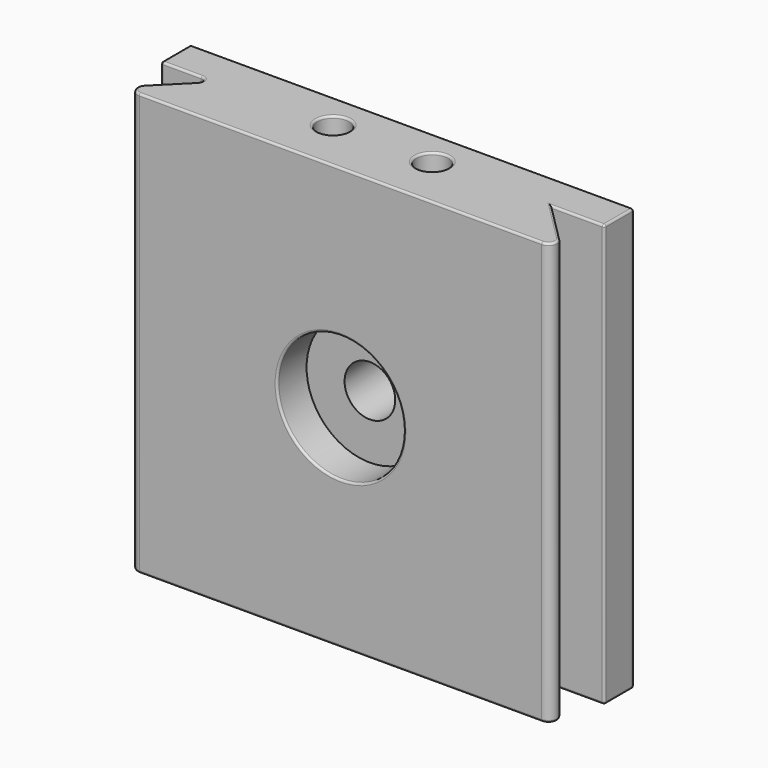
from build123d import *

# Parameters (mm, degrees)
F0_R     = 1.5
F1_DEPTH = 40
F2_R     = 2.4
F3_DEPTH = 8.001
F2_R_2   = 6
F4_DEPTH = 3.48
F5_DEPTH = 0.5
F6_R     = 0.8
F7_R     = 0.5
F8_R     = 0.2


# Not quite as in the source:
# - a feature names something its author has since deleted; it is built from what else it names


with BuildPart() as f1:
    # F0 (on Top) → F1 (new body)
    with BuildSketch(Plane.XY):
        Polygon((-13.1589230299, 2.7048220783), (-21.1589230299, 2.7048220783), (-21.1589230299, -0.2951779217), (-16.1589230299, -0.2951779217), (-21.1589230299, -5.2951779217), (-0.1589230299, -5.2951779217), (20.8410769701, -5.2951779217), (15.8410769701, -0.2951779217), (20.8410769701, -0.2951779217), (20.8410769701, 2.7048220783), (12.8410769701, 2.7048220783), (-0.1589230299, 2.7048220783), align=None)
        with Locations((-4.8589230299, -0.2951779217)):
            Circle(F0_R, mode=Mode.SUBTRACT)
        with BuildLine():
            ThreePointArc((6.0410769701, -0.2951779217), (5.6017371419, -1.3558380934), (4.5410769701, -1.7951779217))
            ThreePointArc((4.5410769701, -1.7951779217), (3.4804167983, 0.7654822501), (6.0410769701, -0.2951779217))
        make_face(mode=Mode.SUBTRACT)
    extrude(amount=F1_DEPTH)

    # F2 (on face) → F3 (cut, through all)
    with BuildSketch(Plane.XZ.offset(5.2951779217)):
        with Locations((-0.1589225605, 19.999999553)):
            Circle(F2_R)
    extrude(amount=-F3_DEPTH, mode=Mode.SUBTRACT)

    # F2 (on face) → F4 (cut)
    with BuildSketch(Plane.XZ.offset(5.2951779217)):
        with Locations((-0.1589225605, 19.999999553)):
            Circle(F2_R_2)
        with Locations((-0.1589225605, 19.999999553)):
            Circle(F2_R, mode=Mode.SUBTRACT)
    extrude(amount=-F4_DEPTH, mode=Mode.SUBTRACT)

    # F5 (add): a face of the model
    f5_faces = [f1.faces().sort_by_distance(p)[0] for p in [
        (20.2610769701, 2.7048220783, 20),
    ]]
    extrude(f5_faces, amount=F5_DEPTH)

    # F6
    f6_edges = [f1.edges().sort_by_distance(p)[0] for p in [
        (20.841077, -5.295178, 20),
        (-21.158923, -5.295178, 20),
    ]]
    fillet(f6_edges, radius=F6_R)

    # F7
    f7_edges = [f1.edges().sort_by_distance(p)[0] for p in [
        (-16.158923, -0.295178, 20),
    ]]
    fillet(f7_edges, radius=F7_R)

    # F8
    f8_edges = [f1.edges().sort_by_distance(p)[0] for p in [
        (-18.402857, -2.539112, 40),
        (-16.90409, -0.603836, 40),
        (-19.966656, -4.801325, 40),
        (-19.262476, -0.295178, 40),
        (-0.158923, -5.295178, 40),
        (-21.158923, 1.454822, 40),
        (19.64881, -4.801325, 40),
        (-0.158923, 3.204822, 40),
        (17.658234, -2.112335, 40),
        (20.841077, 1.454822, 40),
        (18.341077, -0.295178, 40),
        (-6.358923, -0.295178, 40),
        (4.541077, 1.204822, 40),
        (-18.402857, -2.539112, 0),
        (-16.90409, -0.603836, 0),
        (-19.966656, -4.801325, 0),
        (-19.262476, -0.295178, 0),
        (-0.158923, -5.295178, 0),
        (-21.158923, 1.454822, 0),
        (19.64881, -4.801325, 0),
        (-0.158923, 3.204822, 0),
        (17.658234, -2.112335, 0),
        (20.841077, 1.454822, 0),
        (18.341077, -0.295178, 0),
        (-6.358923, -0.295178, 0),
        (4.541077, 1.204822, 0),
        (20.841077, 3.204822, 20),
        (-21.158923, 3.204822, 20),
        (-2.558923, 3.204822, 20),
        (-6.158923, -5.295178, 20),
        (-21.158923, -0.295178, 20),
        (20.841077, -0.295178, 20),
    ]]
    fillet(f8_edges, radius=F8_R)


solid = f1.part
